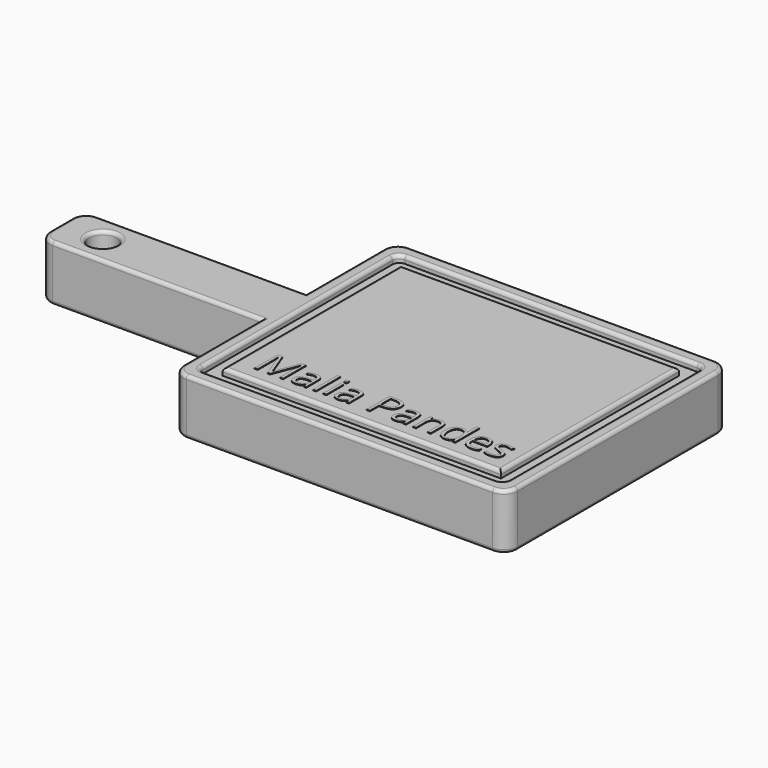
from build123d import *

# Parameters (mm, degrees)
F0_W          = 203.2
F0_H          = 50.8
F1_DEPTH      = 25.4
F2_R          = 12.7
F3_DEPTH      = 25.4
F4_DEPTH      = 25.4
F5_W          = 279.4
F5_H          = 228.6
F5_W_2        = 254
F5_H_2        = 203.2
F6_DEPTH      = 6.35
F7_R          = 6.35
F8_R          = 12.7
F9_R          = 3.175
F10_TEXT_SIZE = 36.7376456408
F11_DEPTH     = 0.508


# Not quite as in the source:
# - Text() gives the source's letters only with a copy of the font that has no kerning and outlines rounded to 1/6400 em; it was checked with that copy


with BuildPart() as f1:
    # F0 (on Top) → F1 (new body)
    with BuildSketch(Plane.XY):
        with Locations((-101.6, 127)):
            Rectangle(F0_W, F0_H)
        Polygon((0, 101.6), (0, 0), (304.8, 0), (304.8, 254), (0, 254), (0, 152.4), align=None)
    extrude(amount=F1_DEPTH)

    # F2 (on face) → F3 (join)
    with BuildSketch(Plane.XY.offset(25.4)):
        Polygon((-203.2, 152.4), (-203.2, 101.6), (0, 101.6), (0, 0), (304.8, 0), (304.8, 254), (0, 254), (0, 152.4), align=None)
        with Locations((-165.1, 127)):
            Circle(F2_R, mode=Mode.SUBTRACT)
    extrude(amount=F3_DEPTH)

    # F2 (on face) → F4 (cut)
    with BuildSketch(Plane.XY.offset(25.4)):
        with Locations((-165.1, 127)):
            Circle(F2_R)
    extrude(amount=-F4_DEPTH, mode=Mode.SUBTRACT)

    # F5 (on face) → F6 (cut)
    with BuildSketch(Plane.XY.offset(50.8)):
        with Locations((152.4, 127)):
            Rectangle(F5_W, F5_H)
        with Locations((152.4, 127)):
            Rectangle(F5_W_2, F5_H_2, mode=Mode.SUBTRACT)
    extrude(amount=-F6_DEPTH, mode=Mode.SUBTRACT)

    # F7
    f7_edges = [f1.edges().sort_by_distance(p)[0] for p in [
        (12.7, 241.3, 47.625),
        (292.1, 12.7, 47.625),
        (12.7, 12.7, 47.625),
        (292.1, 241.3, 47.625),
    ]]
    fillet(f7_edges, radius=F7_R)

    # F8
    f8_edges = [f1.edges().sort_by_distance(p)[0] for p in [
        (0, 0, 25.4),
        (304.8, 254, 25.4),
        (0, 254, 25.4),
        (304.8, 0, 25.4),
        (-203.2, 152.4, 25.4),
        (-203.2, 101.6, 25.4),
    ]]
    fillet(f8_edges, radius=F8_R)

    # F9
    f9_edges = [f1.edges().sort_by_distance(p)[0] for p in [
        (25.4, 127, 50.8),
        (152.4, 228.6, 50.8),
        (279.4, 127, 50.8),
        (152.4, 25.4, 50.8),
        (-203.2, 127, 50.8),
        (-199.480256, 148.680256, 50.8),
        (-199.480256, 105.319744, 50.8),
        (-95.25, 152.4, 50.8),
        (-95.25, 101.6, 50.8),
        (0, 196.85, 50.8),
        (0, 57.15, 50.8),
        (3.719744, 250.280256, 50.8),
        (3.719744, 3.719744, 50.8),
        (152.4, 254, 50.8),
        (152.4, 0, 50.8),
        (301.080256, 250.280256, 50.8),
        (301.080256, 3.719744, 50.8),
        (304.8, 127, 50.8),
        (152.4, 241.3, 50.8),
        (290.240128, 239.440128, 50.8),
        (14.559872, 239.440128, 50.8),
        (292.1, 127, 50.8),
        (12.7, 127, 50.8),
        (290.240128, 14.559872, 50.8),
        (14.559872, 14.559872, 50.8),
        (152.4, 12.7, 50.8),
        (-177.8, 127, 50.8),
        (-95.25, 101.6, 0),
        (-199.480256, 105.319744, 0),
        (0, 57.15, 0),
        (-203.2, 127, 0),
        (3.719744, 3.719744, 0),
        (-199.480256, 148.680256, 0),
        (152.4, 0, 0),
        (-95.25, 152.4, 0),
        (301.080256, 3.719744, 0),
        (0, 196.85, 0),
        (304.8, 127, 0),
        (3.719744, 250.280256, 0),
        (301.080256, 250.280256, 0),
        (152.4, 254, 0),
        (-177.8, 127, 0),
    ]]
    fillet(f9_edges, radius=F9_R)

    # F10 (on face) → F11 (join)
    with BuildSketch(Plane.XY.offset(50.8)):
        with Locations((40.6280712054, 38.5071047148)):
            Text('Malia Pandes', F10_TEXT_SIZE, font='Open Sans', text_align=(TextAlign.LEFT, TextAlign.BOTTOM))
    extrude(amount=F11_DEPTH)


solid = f1.part
